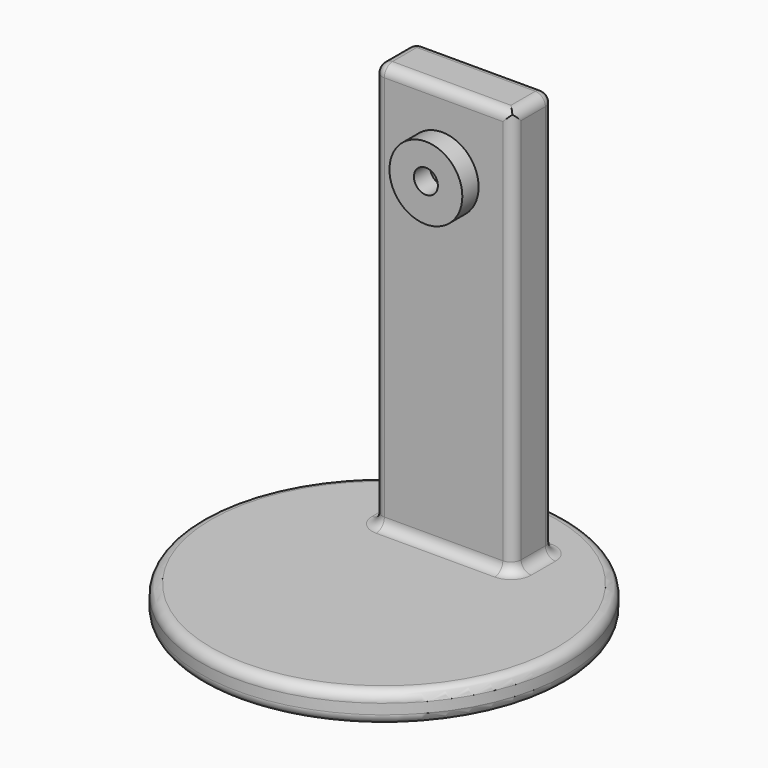
from build123d import *

# Parameters (mm, degrees)
F0_R          = 90
F1_DEPTH      = 15
F3_W          = 68.1982785463
F3_H          = 24.9051749706
F4_DEPTH      = 200
F6_R          = 17.9109144278
F6_R_2        = 5.8846273737
F7_DEPTH      = 10
F8_R          = 5
F9_R          = 5
F10_R         = 5
F11_T1_DEPTH  = 195
F11_T3_DEPTH  = 14.9051749706
F11_T5_DEPTH  = 27.4051749706
F11_T7_DEPTH  = 58.1982785463
F11_S11_W     = 5.1
F11_S11_H     = 5.1
F11_T12_DEPTH = 5.1
F11_S17_W     = 5.1
F11_S17_H     = 5.1
F11_T18_DEPTH = 5.1
F11_T22_ANGLE = 90
F11_T23_DEPTH = 14.9051749706
F11_T25_DEPTH = 58.1982785463
F11_T28_ANGLE = 90
F11_T30_ANGLE = 90
F11_T32_ANGLE = 90
F11_T34_ANGLE = 90


# Not quite as in the source:
# - a fillet or chamfer that OpenCascade refuses, or shapes differently, is made with other operations: its cross-section is extruded or revolved along the edge and cut away or added


with BuildPart() as f1:
    # F0 (on Top) → F1 (new body)
    with BuildSketch(Plane.XY):
        Circle(F0_R)
    extrude(amount=F1_DEPTH)

    # F3 (on face) → F4 (join)
    with BuildSketch(Plane.XY.offset(15)):
        with Locations((0.6982758641, 48.1810383499)):
            Rectangle(F3_W, F3_H)
    extrude(amount=F4_DEPTH)

    # F8
    f8_edges = [f1.edges().sort_by_distance(p)[0] for p in [
        (-90, 0, 15),
    ]]
    fillet(f8_edges, radius=F8_R)

    # F9
    f9_edges = [f1.edges().sort_by_distance(p)[0] for p in [
        (-90, 0, 0),
    ]]
    fillet(f9_edges, radius=F9_R)

    # F10
    f10_edges = [f1.edges().sort_by_distance(p)[0] for p in [
        (0.698276, 35.728451, 215),
        (34.797415, 35.728451, 115),
    ]]
    fillet(f10_edges, radius=F10_R)

    # F11: fillet of radius 5 on 14 edges, made by hand

    # F11_s2 → F11_t1 (cut)
    with BuildSketch(Plane.XY.offset(15)):
        with BuildLine():
            ThreePointArc((-28.400863409, 35.7284508646), (-31.936397315, 37.1929169586), (-33.400863409, 40.7284508646))
            Line((-33.400863409, 40.7284508646), (-33.400863409, 35.7284508646))
            Line((-33.400863409, 35.7284508646), (-28.400863409, 35.7284508646))
        make_face()
        with BuildLine():
            ThreePointArc((-33.400863409, 55.6336258352), (-31.936397315, 59.1691597411), (-28.400863409, 60.6336258352))
            Line((-28.400863409, 60.6336258352), (-33.400863409, 60.6336258352))
            Line((-33.400863409, 60.6336258352), (-33.400863409, 55.6336258352))
        make_face()
        with BuildLine():
            ThreePointArc((34.7974151373, 55.6336258352), (33.3329490432, 59.1691597411), (29.7974151373, 60.6336258352))
            Line((29.7974151373, 60.6336258352), (34.7974151373, 60.6336258352))
            Line((34.7974151373, 60.6336258352), (34.7974151373, 55.6336258352))
        make_face()
    extrude(amount=F11_T1_DEPTH, mode=Mode.SUBTRACT)

    # F11_s4 → F11_t3 (cut)
    with BuildSketch(Plane.XZ.offset(-55.6336258352)):
        with BuildLine():
            ThreePointArc((-33.400863409, 210), (-31.936397315, 213.5355339059), (-28.400863409, 215))
            Line((-28.400863409, 215), (-33.400863409, 215))
            Line((-33.400863409, 215), (-33.400863409, 210))
        make_face()
    extrude(amount=F11_T3_DEPTH, mode=Mode.SUBTRACT)

    # F11_s6 → F11_t5 (cut)
    with BuildSketch(Plane.XZ.offset(-55.6336258352)):
        with BuildLine():
            ThreePointArc((34.7974151373, 210), (33.3329490432, 213.5355339059), (29.7974151373, 215))
            Line((29.7974151373, 215), (34.7974151373, 215))
            Line((34.7974151373, 215), (34.7974151373, 210))
        make_face()
    extrude(amount=F11_T5_DEPTH, mode=Mode.SUBTRACT)

    # F11_s8 → F11_t7 (cut)
    with BuildSketch(Plane.YZ.offset(-28.400863409)):
        with BuildLine():
            ThreePointArc((60.6336258352, 210), (59.1691597411, 213.5355339059), (55.6336258352, 215))
            Line((55.6336258352, 215), (60.6336258352, 215))
            Line((60.6336258352, 215), (60.6336258352, 210))
        make_face()
    extrude(amount=F11_T7_DEPTH, mode=Mode.SUBTRACT)


with BuildPart() as f7:
    # F6 (on face) → F7 (new body)
    with BuildSketch(Plane.XZ.offset(-35.7284508646)):
        with Locations((0, 177.8125017881)):
            Circle(F6_R)
        with Locations((0, 178.5624921322)):
            Circle(F6_R_2, mode=Mode.SUBTRACT)
    extrude(amount=F7_DEPTH)


with BuildPart() as f11_tool10:
    # F11_s11 → F11_t12 (new body)
    with BuildSketch(Plane.XY.offset(210)):
        with Locations((-30.950863409, 58.1836258352)):
            Rectangle(F11_S11_W, F11_S11_H)
    extrude(amount=F11_T12_DEPTH)

    # F11_s13 → F11_t14 (revolve, cut)
    with BuildSketch(Plane(origin=(-28.400863409, 55.6336258352, 210), x_dir=(0.7071067812, -0.7071067812, 0), z_dir=(-0.7071067812, -0.7071067812, 0))):
        with BuildLine():
            ThreePointArc((0, -5), (5, 0), (0, 5))
            Line((0, 5), (0, -5))
        make_face()
    revolve(axis=Axis((-28.400863409, 55.6336258352, 210), (0, 0, 1)), mode=Mode.SUBTRACT)


with BuildPart() as f1_1:
    add(f1.part)

    # F11_t9: cut F11_tool10
    add(f11_tool10.part, mode=Mode.SUBTRACT)


with BuildPart() as f11_tool16:
    # F11_s17 → F11_t18 (new body)
    with BuildSketch(Plane.XY.offset(210)):
        with Locations((32.3474151373, 58.1836258352)):
            Rectangle(F11_S17_W, F11_S17_H)
    extrude(amount=F11_T18_DEPTH)

    # F11_s19 → F11_t20 (revolve, cut)
    with BuildSketch(Plane(origin=(29.7974151373, 55.6336258352, 210), x_dir=(-0.7071067812, -0.7071067812, 0), z_dir=(-0.7071067812, 0.7071067812, 0))):
        with BuildLine():
            ThreePointArc((0, -5), (5, 0), (0, 5))
            Line((0, 5), (0, -5))
        make_face()
    revolve(axis=Axis((29.7974151373, 55.6336258352, 210), (0, 0, 1)), mode=Mode.SUBTRACT)


with BuildPart() as f1_2:
    add(f1_1.part)

    # F11_t15: cut F11_tool16
    add(f11_tool16.part, mode=Mode.SUBTRACT)

    # F11_s21 → F11_t22 (revolve, cut)
    with BuildSketch(Plane.XY.offset(210)):
        with BuildLine():
            ThreePointArc((-33.400863409, 40.7284508646), (-31.936397315, 37.1929169586), (-28.400863409, 35.7284508646))
            Line((-28.400863409, 35.7284508646), (-33.400863409, 35.7284508646))
            Line((-33.400863409, 35.7284508646), (-33.400863409, 40.7284508646))
        make_face()
    revolve(axis=Axis((-33.400863409, 40.7284508646, 210), (-1, 0, 0)), revolution_arc=F11_T22_ANGLE, mode=Mode.SUBTRACT)

    # F11_s24 → F11_t23 (join)
    with BuildSketch(Plane.XZ.offset(-55.6336258352)):
        with BuildLine():
            ThreePointArc((-38.400863409, 15), (-34.8653295031, 16.4644660941), (-33.400863409, 20))
            Line((-33.400863409, 20), (-33.400863409, 15))
            Line((-33.400863409, 15), (-38.400863409, 15))
        make_face()
        with BuildLine():
            ThreePointArc((39.7974151373, 15), (36.2618812314, 16.4644660941), (34.7974151373, 20))
            Line((34.7974151373, 20), (34.7974151373, 15))
            Line((34.7974151373, 15), (39.7974151373, 15))
        make_face()
    extrude(amount=F11_T23_DEPTH)

    # F11_s26 → F11_t25 (join)
    with BuildSketch(Plane.YZ.offset(-28.400863409)):
        with BuildLine():
            ThreePointArc((65.6336258352, 15), (62.0980919292, 16.4644660941), (60.6336258352, 20))
            Line((60.6336258352, 20), (60.6336258352, 15))
            Line((60.6336258352, 15), (65.6336258352, 15))
        make_face()
        with BuildLine():
            ThreePointArc((30.7284508646, 15), (34.2639847705, 16.4644660941), (35.7284508646, 20))
            Line((35.7284508646, 20), (35.7284508646, 15))
            Line((35.7284508646, 15), (30.7284508646, 15))
        make_face()
    extrude(amount=F11_T25_DEPTH)

    # F11_s27 → F11_t28 (revolve)
    with BuildSketch(Plane.YZ.offset(29.7974151373)):
        with BuildLine():
            ThreePointArc((30.7284508646, 15), (34.2639847705, 16.4644660941), (35.7284508646, 20))
            Line((35.7284508646, 20), (35.7284508646, 15))
            Line((35.7284508646, 15), (30.7284508646, 15))
        make_face()
    revolve(axis=Axis((29.7974151373, 40.7284508646, 15), (0, 0, 1)), revolution_arc=F11_T28_ANGLE)

    # F11_s29 → F11_t30 (revolve)
    with BuildSketch(Plane.YZ.offset(-28.400863409)):
        with BuildLine():
            ThreePointArc((30.7284508646, 15), (34.2639847705, 16.4644660941), (35.7284508646, 20))
            Line((35.7284508646, 20), (35.7284508646, 15))
            Line((35.7284508646, 15), (30.7284508646, 15))
        make_face()
    revolve(axis=Axis((-28.400863409, 40.7284508646, 15), (0, 0, -1)), revolution_arc=F11_T30_ANGLE)

    # F11_s31 → F11_t32 (revolve)
    with BuildSketch(Plane.XZ.offset(-55.6336258352)):
        with BuildLine():
            ThreePointArc((39.7974151373, 15), (36.2618812314, 16.4644660941), (34.7974151373, 20))
            Line((34.7974151373, 20), (34.7974151373, 15))
            Line((34.7974151373, 15), (39.7974151373, 15))
        make_face()
    revolve(axis=Axis((29.7974151373, 55.6336258352, 15), (0, 0, 1)), revolution_arc=F11_T32_ANGLE)

    # F11_s33 → F11_t34 (revolve)
    with BuildSketch(Plane.XZ.offset(-55.6336258352)):
        with BuildLine():
            ThreePointArc((-38.400863409, 15), (-34.8653295031, 16.4644660941), (-33.400863409, 20))
            Line((-33.400863409, 20), (-33.400863409, 15))
            Line((-33.400863409, 15), (-38.400863409, 15))
        make_face()
    revolve(axis=Axis((-28.400863409, 55.6336258352, 15), (0, 0, -1)), revolution_arc=F11_T34_ANGLE)


solid = Compound([f7.part, f1_2.part])
